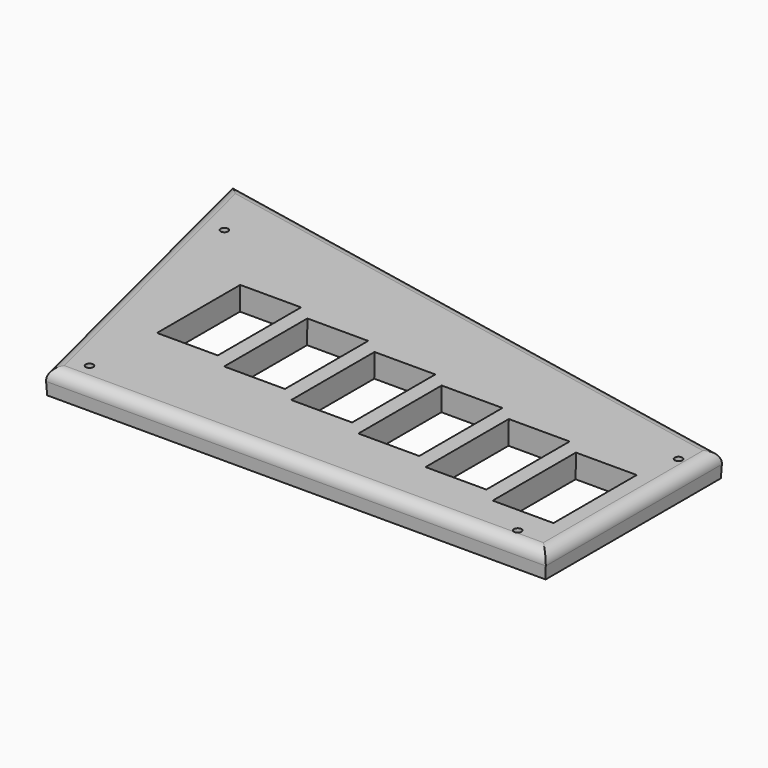
from build123d import *

# Parameters (mm, degrees)
F0_R        = 1.75
F0_W        = 22
F0_H        = 37
F1_DEPTH    = 8.5
F1_TAPER    = -3
F2_DEPTH    = 4.5
F3_T1_DEPTH = 142.1271805444
F3_T3_DEPTH = 228.1816697632
F3_T5_DEPTH = 194.8691049092
F3_T7_DEPTH = 97.8862114568


# Not quite as in the source:
# - a fillet or chamfer that OpenCascade refuses, or shapes differently, is made with other operations: its cross-section is extruded or revolved along the edge and cut away or added


with BuildPart() as f1:
    # F0 (on Top) → F1 (new body)
    with BuildSketch(Plane.XY):
        with BuildLine():
            ThreePointArc((-85.7353818111, -46.3140564233), (-82.1998275149, -55.281625252), (-72.882363358, -52.811342563))
            Line((-72.882363358, -52.811342563), (-84.115426434, -52.811342563))
            Line((-84.115426434, -52.811342563), (-85.7353818111, -46.3140564233))
        make_face()
        with BuildLine():
            Line((-84.115426434, -52.811342563), (-72.882363358, -52.811342563))
            ThreePointArc((-72.882363358, -52.811342563), (-71.9863977223, -50.8998795502), (-71.6790566692, -48.811342563))
            ThreePointArc((-71.6790566692, -48.811342563), (-77.6608605642, -41.6731229923), (-85.7353818111, -46.3140564233))
            Line((-85.7353818111, -46.3140564233), (-84.115426434, -52.811342563))
        make_face()
        with Locations((-78.9290566692, -48.811342563)):
            Circle(F0_R, mode=Mode.SUBTRACT)
        with BuildLine():
            ThreePointArc((73.5070839924, -52.811342563), (72.0709433308, -53.561342563), (70.6348026691, -52.811342563))
            Line((70.6348026691, -52.811342563), (64.8902400226, -52.811342563))
            ThreePointArc((64.8902400226, -52.811342563), (65.5417323383, -54.9628348787), (66.8209433308, -56.811342563))
            Line((66.8209433308, -56.811342563), (77.3209433308, -56.811342563))
            ThreePointArc((77.3209433308, -56.811342563), (78.6001543232, -54.9628348787), (79.2516466389, -52.811342563))
            Line((79.2516466389, -52.811342563), (73.5070839924, -52.811342563))
        make_face()
        with BuildLine():
            ThreePointArc((70.6348026691, -52.811342563), (71.5468947442, -50.1416500527), (73.8209433308, -51.811342563))
            ThreePointArc((73.8209433308, -51.811342563), (73.7406358411, -52.3353911496), (73.5070839924, -52.811342563))
            Line((73.5070839924, -52.811342563), (79.2516466389, -52.811342563))
            ThreePointArc((79.2516466389, -52.811342563), (79.3035984098, -52.3125416331), (79.3209433308, -51.811342563))
            ThreePointArc((79.3209433308, -51.811342563), (71.5697442607, -44.578687484), (64.8902400226, -52.811342563))
            Line((64.8902400226, -52.811342563), (70.6348026691, -52.811342563))
        make_face()
        with BuildLine():
            ThreePointArc((81.75943106, 15.1902968563), (72.6280630891, 8.188657437), (81.75943106, 1.1870180177))
            Line((81.75943106, 1.1870180177), (81.75943106, 15.1902968563))
        make_face()
        with Locations((79.8780630891, 8.188657437)):
            Circle(F0_R, mode=Mode.SUBTRACT)
        with BuildLine():
            Line((81.75943106, 15.1902968563), (81.75943106, 1.1870180177))
            ThreePointArc((81.75943106, 1.1870180177), (83.9978435057, 2.2229295418), (85.75943106, 3.9493165931))
            Line((85.75943106, 3.9493165931), (85.75943106, 12.4279982809))
            ThreePointArc((85.75943106, 12.4279982809), (83.9978435057, 14.1543853322), (81.75943106, 15.1902968563))
        make_face()
        with BuildLine():
            Line((-107.4844802754, 40.9168130189), (-104.4029422618, 28.5574391079))
            ThreePointArc((-104.4029422618, 28.5574391079), (-95.700189339, 28.6381178265), (-91.3719369109, 36.188657437))
            ThreePointArc((-91.3719369109, 36.188657437), (-97.6581749945, 44.5846313066), (-107.4844802754, 40.9168130189))
        make_face()
        with Locations((-100.1219369109, 36.188657437)):
            Circle(F0_R, mode=Mode.SUBTRACT)
        with BuildLine():
            ThreePointArc((-107.4844802754, 40.9168130189), (-108.6120245158, 34.0718408505), (-104.4029422618, 28.5574391079))
            Line((-104.4029422618, 28.5574391079), (-107.4844802754, 40.9168130189))
        make_face()
        with BuildLine():
            ThreePointArc((66.8209433308, -56.811342563), (65.5417323383, -54.9628348787), (64.8902400226, -52.811342563))
            Line((64.8902400226, -52.811342563), (-72.882363358, -52.811342563))
            ThreePointArc((-72.882363358, -52.811342563), (-82.1998275149, -55.281625252), (-85.7353818111, -46.3140564233))
            Line((-85.7353818111, -46.3140564233), (-104.4029422618, 28.5574391079))
            ThreePointArc((-104.4029422618, 28.5574391079), (-108.6120245158, 34.0718408505), (-107.4844802754, 40.9168130189))
            Line((-107.4844802754, 40.9168130189), (-110.8617073408, 54.4621309411))
            Line((-110.8617073408, 54.4621309411), (81.75943106, 15.9099091088))
            Line((81.75943106, 15.9099091088), (81.75943106, 15.1902968563))
            ThreePointArc((81.75943106, 15.1902968563), (83.9978435057, 14.1543853322), (85.75943106, 12.4279982809))
            Line((85.75943106, 12.4279982809), (85.75943106, 19.188657437))
            Line((85.75943106, 19.188657437), (-116.2711964119, 59.6241445901))
            Line((-116.2711964119, 59.6241445901), (-87.24056894, -56.811342563))
            Line((-87.24056894, -56.811342563), (66.8209433308, -56.811342563))
        make_face()
        with BuildLine():
            Line((81.75943106, -52.811342563), (79.2516466389, -52.811342563))
            ThreePointArc((79.2516466389, -52.811342563), (78.6001543232, -54.9628348787), (77.3209433308, -56.811342563))
            Line((77.3209433308, -56.811342563), (85.75943106, -56.811342563))
            Line((85.75943106, -56.811342563), (85.75943106, 3.9493165931))
            ThreePointArc((85.75943106, 3.9493165931), (83.9978435057, 2.2229295418), (81.75943106, 1.1870180177))
            Line((81.75943106, 1.1870180177), (81.75943106, -52.811342563))
        make_face()
        with BuildLine():
            Line((-72.882363358, -52.811342563), (64.8902400226, -52.811342563))
            ThreePointArc((64.8902400226, -52.811342563), (71.5697442607, -44.578687484), (79.3209433308, -51.811342563))
            ThreePointArc((79.3209433308, -51.811342563), (79.3035984098, -52.3125416331), (79.2516466389, -52.811342563))
            Line((79.2516466389, -52.811342563), (81.75943106, -52.811342563))
            Line((81.75943106, -52.811342563), (81.75943106, 1.1870180177))
            ThreePointArc((81.75943106, 1.1870180177), (72.6280630891, 8.188657437), (81.75943106, 15.1902968563))
            Line((81.75943106, 15.1902968563), (81.75943106, 15.9099091088))
            Line((81.75943106, 15.9099091088), (-110.8617073408, 54.4621309411))
            Line((-110.8617073408, 54.4621309411), (-107.4844802754, 40.9168130189))
            ThreePointArc((-107.4844802754, 40.9168130189), (-97.6581749945, 44.5846313066), (-91.3719369109, 36.188657437))
            ThreePointArc((-91.3719369109, 36.188657437), (-95.700189339, 28.6381178265), (-104.4029422618, 28.5574391079))
            Line((-104.4029422618, 28.5574391079), (-85.7353818111, -46.3140564233))
            ThreePointArc((-85.7353818111, -46.3140564233), (-77.6608605642, -41.6731229923), (-71.6790566692, -48.811342563))
            ThreePointArc((-71.6790566692, -48.811342563), (-71.9863977223, -50.8998795502), (-72.882363358, -52.811342563))
        make_face()
        with Locations((-66.1195590496, -4.311342563)):
            Rectangle(F0_W, F0_H, mode=Mode.SUBTRACT)
        with Locations((-39.6195590496, -8.311342563)):
            Rectangle(F0_W, F0_H, mode=Mode.SUBTRACT)
        with Locations((13.3804409504, -16.311342563)):
            Rectangle(F0_W, F0_H, mode=Mode.SUBTRACT)
        with Locations((-13.1195590496, -12.311342563)):
            Rectangle(F0_W, F0_H, mode=Mode.SUBTRACT)
        with Locations((39.8804409504, -20.311342563)):
            Rectangle(F0_W, F0_H, mode=Mode.SUBTRACT)
        with Locations((66.3804409504, -24.311342563)):
            Rectangle(F0_W, F0_H, mode=Mode.SUBTRACT)
    extrude(amount=F1_DEPTH, taper=F1_TAPER)

    # F0 (on Top) → F2 (cut)
    with BuildSketch(Plane.XY):
        with BuildLine():
            Line((-72.882363358, -52.811342563), (64.8902400226, -52.811342563))
            ThreePointArc((64.8902400226, -52.811342563), (71.5697442607, -44.578687484), (79.3209433308, -51.811342563))
            ThreePointArc((79.3209433308, -51.811342563), (79.3035984098, -52.3125416331), (79.2516466389, -52.811342563))
            Line((79.2516466389, -52.811342563), (81.75943106, -52.811342563))
            Line((81.75943106, -52.811342563), (81.75943106, 1.1870180177))
            ThreePointArc((81.75943106, 1.1870180177), (72.6280630891, 8.188657437), (81.75943106, 15.1902968563))
            Line((81.75943106, 15.1902968563), (81.75943106, 15.9099091088))
            Line((81.75943106, 15.9099091088), (-110.8617073408, 54.4621309411))
            Line((-110.8617073408, 54.4621309411), (-107.4844802754, 40.9168130189))
            ThreePointArc((-107.4844802754, 40.9168130189), (-97.6581749945, 44.5846313066), (-91.3719369109, 36.188657437))
            ThreePointArc((-91.3719369109, 36.188657437), (-95.700189339, 28.6381178265), (-104.4029422618, 28.5574391079))
            Line((-104.4029422618, 28.5574391079), (-85.7353818111, -46.3140564233))
            ThreePointArc((-85.7353818111, -46.3140564233), (-77.6608605642, -41.6731229923), (-71.6790566692, -48.811342563))
            ThreePointArc((-71.6790566692, -48.811342563), (-71.9863977223, -50.8998795502), (-72.882363358, -52.811342563))
        make_face()
        with Locations((-66.1195590496, -4.311342563)):
            Rectangle(F0_W, F0_H, mode=Mode.SUBTRACT)
        with Locations((-39.6195590496, -8.311342563)):
            Rectangle(F0_W, F0_H, mode=Mode.SUBTRACT)
        with Locations((13.3804409504, -16.311342563)):
            Rectangle(F0_W, F0_H, mode=Mode.SUBTRACT)
        with Locations((-13.1195590496, -12.311342563)):
            Rectangle(F0_W, F0_H, mode=Mode.SUBTRACT)
        with Locations((39.8804409504, -20.311342563)):
            Rectangle(F0_W, F0_H, mode=Mode.SUBTRACT)
        with Locations((66.3804409504, -24.311342563)):
            Rectangle(F0_W, F0_H, mode=Mode.SUBTRACT)
    extrude(amount=F2_DEPTH, mode=Mode.SUBTRACT)

    # F3: fillet of radius 4 on 4 edges, made by hand

    # F3_s2 → F3_t1 (cut)
    with BuildSketch(Plane(origin=(-23.5203588914, 94.3350069914, 0), x_dir=(0, 0, 1), z_dir=(0.2419218956, -0.9702957263, 0))):
        with BuildLine():
            ThreePointArc((4.290656175, 98.6179226466), (7.2534183028, 97.5249019916), (8.5, 94.6234045075))
            Line((8.5, 94.6234045075), (8.5, 98.8385250087))
            Line((8.5, 98.8385250087), (4.290656175, 98.6179226466))
        make_face()
    extrude(amount=F3_T1_DEPTH, mode=Mode.SUBTRACT)

    # F3_s4 → F3_t3 (cut)
    with BuildSketch(Plane(origin=(89.4546965917, -17.9039400119, 0), x_dir=(0, 0, 1), z_dir=(-0.980553261, 0.1962531587, 0))):
        with BuildLine():
            ThreePointArc((4.290656175, 35.8709236176), (7.2534183028, 34.7779029626), (8.5, 31.8764054785))
            Line((8.5, 31.8764054785), (8.5, 36.0915259797))
            Line((8.5, 36.0915259797), (4.290656175, 35.8709236176))
        make_face()
    extrude(amount=F3_T3_DEPTH, mode=Mode.SUBTRACT)

    # F3_s6 → F3_t5 (cut)
    with BuildSketch(Plane.YZ.offset(-98.1264064725)):
        with BuildLine():
            ThreePointArc((-53.0416881858, 8.5), (-55.9431856699, 7.2534183028), (-57.0362063248, 4.290656175))
            Line((-57.0362063248, 4.290656175), (-57.2568086869, 8.5))
            Line((-57.2568086869, 8.5), (-53.0416881858, 8.5))
        make_face()
    extrude(amount=F3_T5_DEPTH, mode=Mode.SUBTRACT)

    # F3_s8 → F3_t7 (cut)
    with BuildSketch(Plane.XZ.offset(-30.091601517)):
        with BuildLine():
            ThreePointArc((81.9897766828, 8.5), (84.8912741668, 7.2534183028), (85.9842948218, 4.290656175))
            Line((85.9842948218, 4.290656175), (86.2048971839, 8.5))
            Line((86.2048971839, 8.5), (81.9897766828, 8.5))
        make_face()
    extrude(amount=F3_T7_DEPTH, mode=Mode.SUBTRACT)


solid = f1.part
